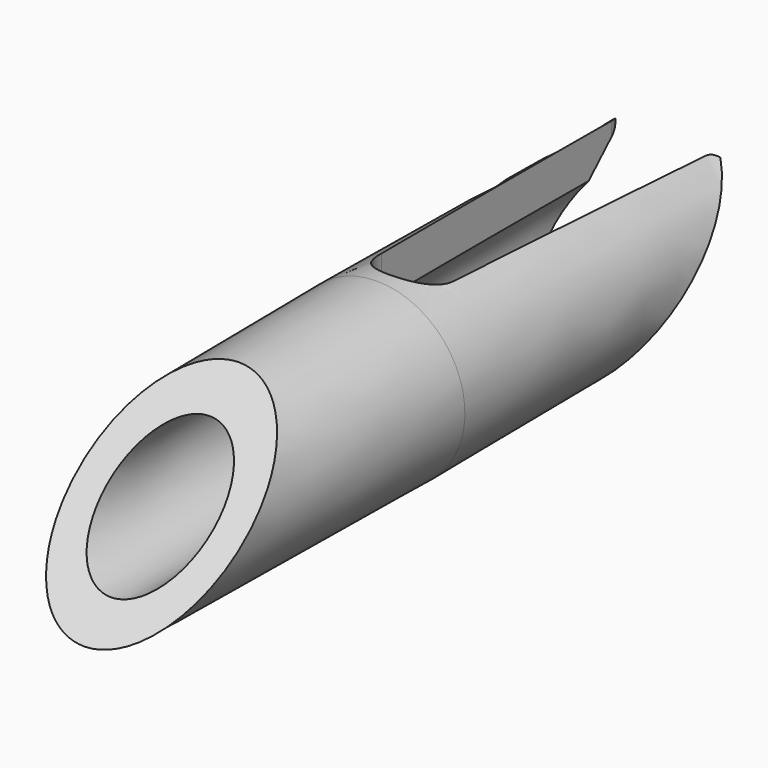
from build123d import *

# Parameters (mm, degrees)
F3_DEPTH = 25
F5_DEPTH = 12.5


# Not quite as in the source:
# - a feature of the source that left no trace in its solid (it failed there, or was rolled back) is left out


with BuildPart() as f1:
    # F0 (on Right) → F1 (revolve)
    with BuildSketch(Plane.YZ):
        Polygon((-1, 2), (0, 2), (1, 2), (1, 3.5723834783), (25, 3.7818283052), (25, 5.7818283052), (0, 6), (-25, 5.7818283052), (-25, 3.7818283052), (-1, 3.5723834783), align=None)
    revolve(axis=Axis((0, 180.1521787086, 0), (0, 1, 0)))

    # F2 (on Top) → F3 (cut)
    with BuildSketch(Plane.XY):
        with BuildLine():
            Line((-3.2170944919, 24.0348994967), (-2.5, 3.5))
            ThreePointArc((-2.5, 3.5), (0, 1), (2.5, 3.5))
            Line((2.5, 3.5), (3.2170944919, 24.0348994967))
            ThreePointArc((3.2170944919, 24.0348994967), (3.5218269484, 24.7193398003), (4.2164853189, 25))
            Line((4.2164853189, 25), (5.7818283052, 25))
            Line((5.7818283052, 25), (5.7818283052, 27.9599502683))
            Line((5.7818283052, 27.9599502683), (-5.9923287481, 27.9599502683))
            Line((-5.9923287481, 27.9599502683), (-5.7818283052, 25))
            Line((-5.7818283052, 25), (-4.2164853189, 25))
            ThreePointArc((-4.2164853189, 25), (-3.5218269484, 24.7193398003), (-3.2170944919, 24.0348994967))
        make_face()
    extrude(amount=F3_DEPTH, mode=Mode.SUBTRACT)

    # F4 (on Right) → F5 (cut, symmetric)
    with BuildSketch(Plane.YZ):
        Polygon((32.3949936356, 6.6679690088), (27.2697879307, 6.7125111288), (9.7397706777, -8.7493574537), (32.3949936356, -8.9470665892), align=None)
        Polygon((-29.6528312787, -5.7412236618), (-25, -5.7818283052), (-3.2005671173, 13.4457606663), (-29.6528312787, 14.9152847007), align=None)
    extrude(amount=F5_DEPTH, both=True, mode=Mode.SUBTRACT)


solid = f1.part
